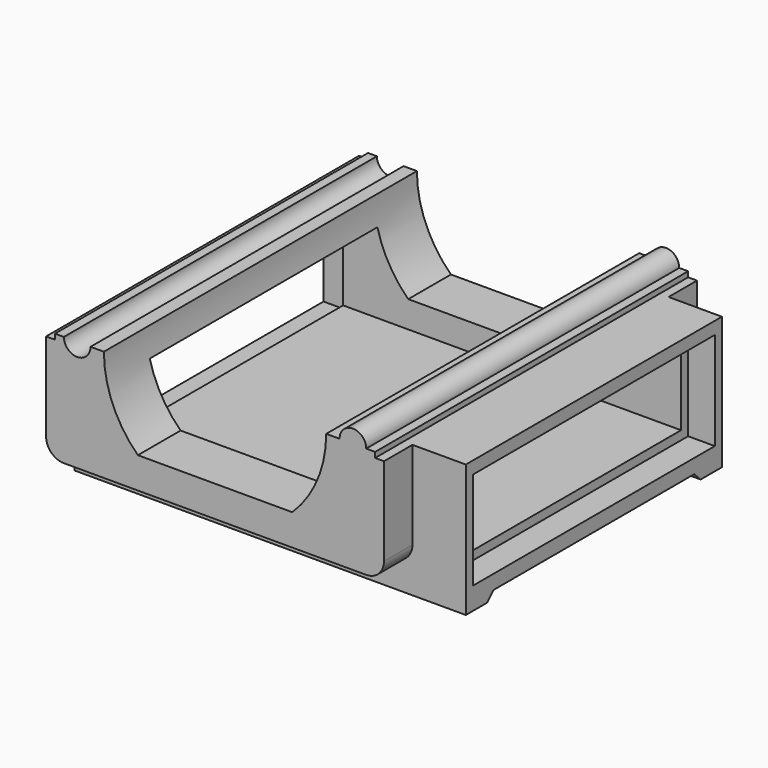
from build123d import *

# Parameters (mm, degrees)
F3_DEPTH     = 22
F0_R         = 4.75
F4_DEPTH     = 25
F2_W         = 6
F2_H         = 3
F5_DEPTH     = 19
F6_W         = 60
F6_H         = 32
F7_DEPTH     = 3
F8_DEPTH     = 3
F9_DEPTH     = 3
F10_DEPTH    = 3
F11_DEPTH    = 6
F12_W        = 34
F12_H        = 11
F12_W_2      = 32
F12_H_2      = 9
F13_DEPTH    = 3
F14_W        = 34
F14_H        = 11
F14_W_2      = 32
F14_H_2      = 9
F15_DEPTH    = 3
F2_W_2       = 4
F16_DEPTH    = 25
F17_T4_DEPTH = 59.4300979278
F17_T9_DEPTH = 59.4300979278
F18_W        = 6
F18_H        = 11.9
F19_DEPTH    = 4
F20_W        = 6
F20_H        = 11.9
F21_DEPTH    = 4
F22_R        = 2


# Not quite as in the source:
# - a fillet or chamfer that OpenCascade refuses, or shapes differently, is made with other operations: its cross-section is extruded or revolved along the edge and cut away or added


with BuildPart() as f3:
    # F1 (on Front) → F3 (new body, symmetric)
    with BuildSketch(Plane.XZ):
        with BuildLine():
            Line((14, 0), (12.5, 0))
            ThreePointArc((12.5, 0), (11.5039872942, -4.8896090165), (8.6746757864, -9))
            Line((8.6746757864, -9), (12.6194294641, -9))
            ThreePointArc((12.6194294641, -9), (14.1666094691, -6.2894495904), (15.139409409, -3.3238957184))
            Line((15.139409409, -3.3238957184), (15.139409409, -1.4560131956))
            ThreePointArc((15.139409409, -1.4560131956), (14.318711321, -0.9244225531), (14, 0))
        make_face()
        with BuildLine():
            Line((8.6746757864, -9), (3.0413812651, -9))
            ThreePointArc((3.0413812651, -9), (0, -9.5), (-3.0413812651, -9))
            Line((-3.0413812651, -9), (-8.6746757864, -9))
            ThreePointArc((-8.6746757864, -9), (0, -12.5), (8.6746757864, -9))
        make_face()
        with BuildLine():
            ThreePointArc((-3.0413812651, -9), (0, -9.5), (3.0413812651, -9))
            Line((3.0413812651, -9), (-3.0413812651, -9))
        make_face()
        with BuildLine():
            Line((12.6194294641, -9), (8.6746757864, -9))
            ThreePointArc((8.6746757864, -9), (0, -12.5), (-8.6746757864, -9))
            Line((-8.6746757864, -9), (-12.6194294641, -9))
            ThreePointArc((-12.6194294641, -9), (-10.9697184602, -10.9505834047), (-9.0220182155, -12.603697367))
            Line((-9.0220182155, -12.603697367), (9.0220182155, -12.603697367))
            ThreePointArc((9.0220182155, -12.603697367), (10.9697184602, -10.9505834047), (12.6194294641, -9))
        make_face()
        with BuildLine():
            ThreePointArc((15.139409409, 1.4560131956), (14.318711321, 0.9244225531), (14, 0))
            Line((14, 0), (15.139409409, 0))
            Line((15.139409409, 0), (15.139409409, 1.4560131956))
        make_face()
        with BuildLine():
            Line((15.139409409, 0), (14, 0))
            ThreePointArc((14, 0), (14.318711321, -0.9244225531), (15.139409409, -1.4560131956))
            Line((15.139409409, -1.4560131956), (15.139409409, 0))
        make_face()
        with BuildLine():
            ThreePointArc((-8.6746757864, -9), (-11.5039872942, -4.8896090165), (-12.5, 0))
            Line((-12.5, 0), (-14, 0))
            ThreePointArc((-14, 0), (-14.318711321, -0.9244225531), (-15.139409409, -1.4560131956))
            Line((-15.139409409, -1.4560131956), (-15.139409409, -3.3238957184))
            ThreePointArc((-15.139409409, -3.3238957184), (-14.1666094691, -6.2894495904), (-12.6194294641, -9))
            Line((-12.6194294641, -9), (-8.6746757864, -9))
        make_face()
        with BuildLine():
            ThreePointArc((15.139409409, -3.3238957184), (14.1666094691, -6.2894495904), (12.6194294641, -9))
            Line((12.6194294641, -9), (15.139409409, -9))
            Line((15.139409409, -9), (15.139409409, -3.3238957184))
        make_face()
        with BuildLine():
            Line((15.139409409, -9), (12.6194294641, -9))
            ThreePointArc((12.6194294641, -9), (10.9697184602, -10.9505834047), (9.0220182155, -12.603697367))
            Line((9.0220182155, -12.603697367), (14.2178343175, -12.603697367))
            ThreePointArc((14.2178343175, -12.603697367), (15.5800609184, -10.8748196205), (16.7332005307, -9))
            Line((16.7332005307, -9), (15.139409409, -9))
        make_face()
        with BuildLine():
            Line((15.5, 0), (15.139409409, 0))
            Line((15.139409409, 0), (15.139409409, -1.4560131956))
            ThreePointArc((15.139409409, -1.4560131956), (15.2823875721, -1.484131002), (15.4274193548, -1.4982429876))
            ThreePointArc((15.4274193548, -1.4982429876), (15.4818442054, -0.75), (15.5, 0))
        make_face()
        with BuildLine():
            Line((15.139409409, 1.4560131956), (15.139409409, 0))
            Line((15.139409409, 0), (15.5, 0))
            ThreePointArc((15.5, 0), (15.4818442054, 0.75), (15.4274193548, 1.4982429876))
            ThreePointArc((15.4274193548, 1.4982429876), (15.2823875721, 1.484131002), (15.139409409, 1.4560131956))
        make_face()
        with BuildLine():
            ThreePointArc((15.4274193548, -1.4982429876), (15.2823875721, -1.484131002), (15.139409409, -1.4560131956))
            Line((15.139409409, -1.4560131956), (15.139409409, -3.3238957184))
            ThreePointArc((15.139409409, -3.3238957184), (15.3106501215, -2.4153659883), (15.4274193548, -1.4982429876))
        make_face()
        with BuildLine():
            ThreePointArc((-9.0220182155, -12.603697367), (-10.9697184602, -10.9505834047), (-12.6194294641, -9))
            Line((-12.6194294641, -9), (-15.139409409, -9))
            Line((-15.139409409, -9), (-16.7332005307, -9))
            ThreePointArc((-16.7332005307, -9), (-15.5800609184, -10.8748196205), (-14.2178343175, -12.603697367))
            Line((-14.2178343175, -12.603697367), (-9.0220182155, -12.603697367))
        make_face()
        with BuildLine():
            Line((-15.139409409, -9), (-12.6194294641, -9))
            ThreePointArc((-12.6194294641, -9), (-14.1666094691, -6.2894495904), (-15.139409409, -3.3238957184))
            Line((-15.139409409, -3.3238957184), (-15.139409409, -9))
        make_face()
        with BuildLine():
            Line((15.139409409, -3.3238957184), (15.139409409, -9))
            Line((15.139409409, -9), (16.7332005307, -9))
            ThreePointArc((16.7332005307, -9), (18.3490087673, -4.9309103884), (18.9905239528, -0.6))
            Line((18.9905239528, -0.6), (18, -0.6))
            Line((18, -0.6), (18, 0))
            Line((18, 0), (17, 0))
            ThreePointArc((17, 0), (16.5346808765, -1.0860181784), (15.4274193548, -1.4982429876))
            ThreePointArc((15.4274193548, -1.4982429876), (15.3106501215, -2.4153659883), (15.139409409, -3.3238957184))
        make_face()
        with BuildLine():
            ThreePointArc((5.1944223175, -14.603697367), (7.1782167254, -13.7376564465), (9.0220182155, -12.603697367))
            Line((9.0220182155, -12.603697367), (-9.0220182155, -12.603697367))
            ThreePointArc((-9.0220182155, -12.603697367), (-7.1782167254, -13.7376564465), (-5.1944223175, -14.603697367))
            Line((-5.1944223175, -14.603697367), (5.1944223175, -14.603697367))
        make_face()
        with BuildLine():
            Line((14.2178343175, -12.603697367), (9.0220182155, -12.603697367))
            ThreePointArc((9.0220182155, -12.603697367), (7.1782167254, -13.7376564465), (5.1944223175, -14.603697367))
            Line((5.1944223175, -14.603697367), (12.1545062924, -14.603697367))
            ThreePointArc((12.1545062924, -14.603697367), (13.2240344567, -13.6427604497), (14.2178343175, -12.603697367))
        make_face()
        with BuildLine():
            Line((17, 0), (15.5, 0))
            ThreePointArc((15.5, 0), (15.4818442054, -0.75), (15.4274193548, -1.4982429876))
            ThreePointArc((15.4274193548, -1.4982429876), (16.5346808765, -1.0860181784), (17, 0))
        make_face()
        with BuildLine():
            ThreePointArc((15.4274193548, 1.4982429876), (15.4818442054, 0.75), (15.5, 0))
            Line((15.5, 0), (17, 0))
            ThreePointArc((17, 0), (16.5346808765, 1.0860181784), (15.4274193548, 1.4982429876))
        make_face()
        with BuildLine():
            Line((-15.139409409, -3.3238957184), (-15.139409409, -1.4560131956))
            ThreePointArc((-15.139409409, -1.4560131956), (-15.2823875721, -1.484131002), (-15.4274193548, -1.4982429876))
            ThreePointArc((-15.4274193548, -1.4982429876), (-15.3106501215, -2.4153659883), (-15.139409409, -3.3238957184))
        make_face()
        with BuildLine():
            Line((-16.7332005307, -9), (-15.139409409, -9))
            Line((-15.139409409, -9), (-15.139409409, -3.3238957184))
            ThreePointArc((-15.139409409, -3.3238957184), (-15.3106501215, -2.4153659883), (-15.4274193548, -1.4982429876))
            ThreePointArc((-15.4274193548, -1.4982429876), (-16.5346808765, -1.0860181784), (-17, 0))
            Line((-17, 0), (-18, 0))
            Line((-18, 0), (-18, -0.6))
            Line((-18, -0.6), (-18.9905239528, -0.6))
            ThreePointArc((-18.9905239528, -0.6), (-18.3490087673, -4.9309103884), (-16.7332005307, -9))
        make_face()
        with BuildLine():
            ThreePointArc((-5.1944223175, -14.603697367), (-7.1782167254, -13.7376564465), (-9.0220182155, -12.603697367))
            Line((-9.0220182155, -12.603697367), (-14.2178343175, -12.603697367))
            ThreePointArc((-14.2178343175, -12.603697367), (-13.2240344567, -13.6427604497), (-12.1545062924, -14.603697367))
            Line((-12.1545062924, -14.603697367), (-5.1944223175, -14.603697367))
        make_face()
        with BuildLine():
            ThreePointArc((18.9905239528, -0.6), (18.3490087673, -4.9309103884), (16.7332005307, -9))
            Line((16.7332005307, -9), (19, -9))
            Line((19, -9), (19, -0.6))
            Line((19, -0.6), (18.9905239528, -0.6))
        make_face()
        with BuildLine():
            Line((19, -9), (16.7332005307, -9))
            ThreePointArc((16.7332005307, -9), (15.5800609184, -10.8748196205), (14.2178343175, -12.603697367))
            Line((14.2178343175, -12.603697367), (19, -12.603697367))
            Line((19, -12.603697367), (19, -9))
        make_face()
        with BuildLine():
            Line((19, -12.603697367), (14.2178343175, -12.603697367))
            ThreePointArc((14.2178343175, -12.603697367), (13.2240344567, -13.6427604497), (12.1545062924, -14.603697367))
            Line((12.1545062924, -14.603697367), (19, -14.603697367))
            Line((19, -14.603697367), (19, -12.603697367))
        make_face()
        with BuildLine():
            ThreePointArc((-14.2178343175, -12.603697367), (-15.5800609184, -10.8748196205), (-16.7332005307, -9))
            Line((-16.7332005307, -9), (-19, -9))
            Line((-19, -9), (-19, -12.603697367))
            Line((-19, -12.603697367), (-14.2178343175, -12.603697367))
        make_face()
        with BuildLine():
            Line((-19, -9), (-16.7332005307, -9))
            ThreePointArc((-16.7332005307, -9), (-18.3490087673, -4.9309103884), (-18.9905239528, -0.6))
            Line((-18.9905239528, -0.6), (-19, -0.6))
            Line((-19, -0.6), (-19, -9))
        make_face()
        with BuildLine():
            ThreePointArc((-12.1545062924, -14.603697367), (-13.2240344567, -13.6427604497), (-14.2178343175, -12.603697367))
            Line((-14.2178343175, -12.603697367), (-19, -12.603697367))
            Line((-19, -12.603697367), (-19, -14.603697367))
            Line((-19, -14.603697367), (-12.1545062924, -14.603697367))
        make_face()
    extrude(amount=F3_DEPTH, both=True)

    # F0 (on Top) → F4 (cut)
    with BuildSketch(Plane.XY):
        with Locations((3, 0)):
            Circle(F0_R)
    extrude(amount=-F4_DEPTH, mode=Mode.SUBTRACT)

    # F2 (on Right) → F5 (join, symmetric)
    with BuildSketch(Plane.YZ):
        with Locations((-15, -14)):
            Rectangle(F2_W, F2_H)
        with Locations((15, -14)):
            Rectangle(F2_W, F2_H)
    extrude(amount=F5_DEPTH, both=True)

    # F6 (on face) → F7 (cut)
    with BuildSketch(Plane.XY.offset(-9)):
        with Locations((3, 0)):
            Rectangle(F6_W, F6_H)
    extrude(amount=-F7_DEPTH, mode=Mode.SUBTRACT)

    # F6 (on face) → F8 (cut)
    with BuildSketch(Plane.XY.offset(-9)):
        with Locations((3, 0)):
            Rectangle(F6_W, F6_H)
    extrude(amount=F8_DEPTH, mode=Mode.SUBTRACT)

    # F9 (cut): a face of the model
    f9_faces = [f3.faces().sort_by_distance(p)[0] for p in [
        (-14.9829280499, 0, -6),
    ]]
    extrude(f9_faces, amount=-F9_DEPTH, mode=Mode.SUBTRACT)

    # F10 (cut): a face of the model
    f10_faces = [f3.faces().sort_by_distance(p)[0] for p in [
        (14.9829280499, 0, -6),
    ]]
    extrude(f10_faces, amount=-F10_DEPTH, mode=Mode.SUBTRACT)

    # F11 (add): a face of the model
    f11_faces = [f3.faces().sort_by_distance(p)[0] for p in [
        (19, 20, -14.1391535047),
    ]]
    extrude(f11_faces, amount=F11_DEPTH)

    # F12 (on face) → F13 (cut)
    with BuildSketch(Plane.YZ.offset(25)):
        with Locations((0, -7.5)):
            Rectangle(F12_W, F12_H)
        with Locations((0, -7.5)):
            Rectangle(F12_W_2, F12_H_2, mode=Mode.SUBTRACT)
    extrude(amount=-F13_DEPTH, mode=Mode.SUBTRACT)

    # F14 (on face) → F15 (cut)
    with BuildSketch(Plane(origin=(-19, 0, 0), x_dir=(0, -1, 0), z_dir=(-1, 0, 0))):
        with Locations((0, -7.5)):
            Rectangle(F14_W, F14_H)
        with Locations((0, -7.5)):
            Rectangle(F14_W_2, F14_H_2, mode=Mode.SUBTRACT)
    extrude(amount=-F15_DEPTH, mode=Mode.SUBTRACT)

    # F2 (on Right) → F16 (cut, symmetric)
    with BuildSketch(Plane.YZ):
        with Locations((20, -14)):
            Rectangle(F2_W_2, F2_H)
        with Locations((-20, -14)):
            Rectangle(F2_W_2, F2_H)
    extrude(amount=F16_DEPTH, both=True, mode=Mode.SUBTRACT)

    # F17: chamfer of 3 on 2 edges, made by hand


with BuildPart() as f17_tool2:
    # F17_s3 → F17_t4 (new body)
    with BuildSketch(Plane.YZ.offset(32.7150489639)):
        Polygon((15, -15.5), (12, -12.5), (12, -15.5), align=None)
    extrude(amount=-F17_T4_DEPTH)

    split(bisect_by=Plane.XY.offset(-14.603697367), keep=Keep.BOTTOM)


with BuildPart() as f3_1:
    add(f3.part)

    # F17_t1: cut F17_tool2
    add(f17_tool2.part, mode=Mode.SUBTRACT)


with BuildPart() as f17_tool7:
    # F17_s8 → F17_t9 (new body)
    with BuildSketch(Plane.YZ.offset(32.7150489639)):
        Polygon((-12, -12.5), (-15, -15.5), (-12, -15.5), align=None)
    extrude(amount=-F17_T9_DEPTH)

    split(bisect_by=Plane.XY.offset(-14.603697367), keep=Keep.BOTTOM)


with BuildPart() as f3_2:
    add(f3_1.part)

    # F17_t6: cut F17_tool7
    add(f17_tool7.part, mode=Mode.SUBTRACT)

    # F18 (on face) → F19 (cut)
    with BuildSketch(Plane.XZ.offset(22)):
        with Locations((22, -6.55)):
            Rectangle(F18_W, F18_H)
    extrude(amount=-F19_DEPTH, mode=Mode.SUBTRACT)

    # F20 (on face) → F21 (cut)
    with BuildSketch(Plane(origin=(0, 22, 0), x_dir=(-1, 0, 0), z_dir=(0, 1, 0))):
        with Locations((-22, -6.55)):
            Rectangle(F20_W, F20_H)
    extrude(amount=-F21_DEPTH, mode=Mode.SUBTRACT)

    # F22
    f22_edges = [f3_2.edges().sort_by_distance(p)[0] for p in [
        (-19, 20, -12.5),
        (19, -20, -12.5),
        (19, 20, -12.5),
        (-19, -20, -12.5),
    ]]
    fillet(f22_edges, radius=F22_R)


solid = f3_2.part
